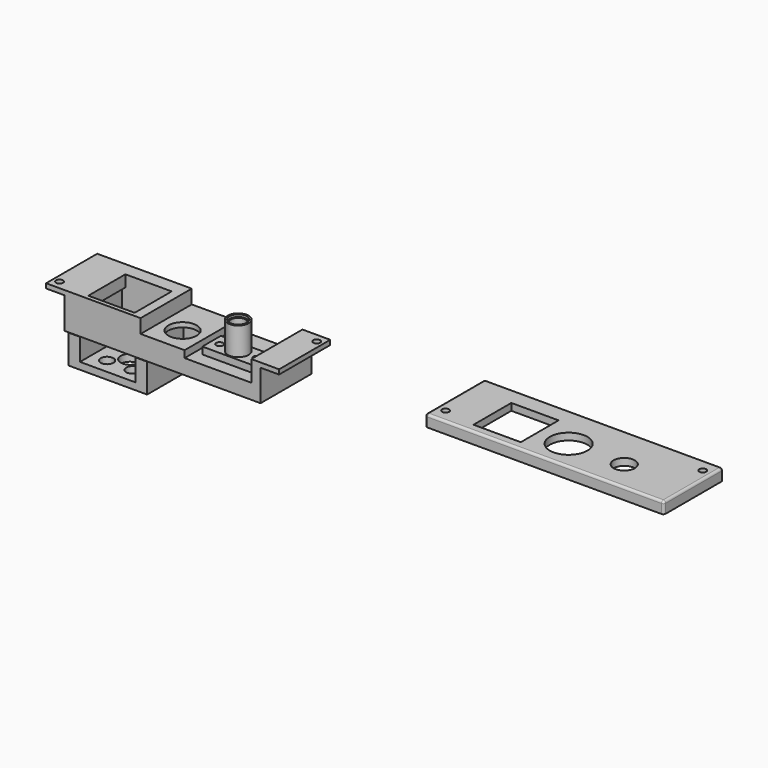
from build123d import *

# Parameters (mm, degrees)
F0_W      = 84.6
F0_H      = 27.6
F0_R      = 1.2
F0_R_2    = 3.1
F1_DEPTH  = 1.5
F2_W      = 103
F2_H      = 32
F2_R      = 1.5
F2_W_2    = 20.4
F2_H_2    = 20.4
F2_R_2    = 8.1
F2_R_3    = 4.6
F3_DEPTH  = 5
F4_W      = 101
F4_H      = 30
F5_DEPTH  = 2
F6_R      = 1
F7_W      = 8
F7_H      = 2
F8_DEPTH  = 27.6
F9_D      = 3
F9_DEPTH  = 5
F9_START  = 8.5
F9_TIP    = 0.9012909285
F10_W     = 23
F10_H     = 10
F10_R     = 1.5
F11_DEPTH = 3
F12_R     = 4.5
F13_DEPTH = 12
F14_R     = 3.1
F15_DEPTH = 25
F16_W     = 19
F16_H     = 27.6
F17_DEPTH = 3
F18_D     = 12.2
F18_DEPTH = 5
F18_TIP   = 3.6652497761
F19_R     = 3.75
F20_DEPTH = 1
F21_W     = 30.8
F21_H     = 9
F21_W_2   = 2
F21_W_3   = 84.6
F21_H_2   = 5
F22_DEPTH = 27.6
F23_W     = 20
F23_H     = 20
F24_DEPTH = 25
F25_W     = 1.5
F25_H     = 20
F26_DEPTH = 10.5
F27_W     = 13
F27_H     = 17
F28_DEPTH = 7.5
F30_W     = 34
F30_H     = 24
F31_DEPTH = 12.5
F32_W     = 24
F32_H     = 9.5
F33_DEPTH = 25
F34_R     = 4
F34_R_2   = 1.6
F34_R_3   = 2.75
F35_DEPTH = 25
F36_R     = 1.2
F37_DEPTH = 8
F38_DEPTH = 25


with BuildPart() as f1:
    # F0 (on Top) → F1 (new body)
    with BuildSketch(Plane.XY):
        Rectangle(F0_W, F0_H)
        with Locations((16, -3)):
            Circle(F0_R, mode=Mode.SUBTRACT)
        with Locations((24, -3)):
            Circle(F0_R_2, mode=Mode.SUBTRACT)
        with Locations((32, -3)):
            Circle(F0_R, mode=Mode.SUBTRACT)
    extrude(amount=F1_DEPTH)

    # F7 (on face) → F8 (join)
    with BuildSketch(Plane.XZ.offset(13.8)):
        Polygon((-42.3, 8.5), (-42.3, 1.5), (-40.3, 1.5), (-40.3, 10.5), (-50.3, 10.5), (-50.3, 8.5), align=None)
        Polygon((42.3, 8.5), (42.3, 10.5), (40.3, 10.5), (40.3, 1.5), (42.3, 1.5), align=None)
        with Locations((46.3, 9.5)):
            Rectangle(F7_W, F7_H)
    extrude(amount=-F8_DEPTH)

    # F9
    # its depths count from where the whole tool has entered the part; down to there all is cleared
    with Locations(Plane(origin=(0, 0, 0), x_dir=(1, 0, 0), z_dir=(0, 0, -1))):
        with Locations((-47.5, 10), (47.5, -10)):
            Hole(F9_D / 2, depth=F9_START)
    with Locations(Plane(origin=(0, 0, 0), x_dir=(1, 0, 0), z_dir=(0, 0, -1)).offset(-F9_START)):
        with Locations((-47.5, 10), (47.5, -10)):
            Hole(F9_D / 2, depth=F9_DEPTH)
            with Locations((0, 0, -(F9_DEPTH + F9_TIP / 2))):  # 118° drill point
                Cone(0, F9_D / 2, F9_TIP, mode=Mode.SUBTRACT)

    # F16 (on face) → F17 (join)
    with BuildSketch(Plane.XY.offset(1.5)):
        Rectangle(F16_W, F16_H)
    extrude(amount=F17_DEPTH)

    # F18
    with Locations(Plane(origin=(0, 0, 0), x_dir=(1, 0, 0), z_dir=(0, 0, -1))):
        with Locations((0, 3)):
            Hole(F18_D / 2, depth=F18_DEPTH)
            with Locations((0, 0, -(F18_DEPTH + F18_TIP / 2))):  # 118° drill point
                Cone(0, F18_D / 2, F18_TIP, mode=Mode.SUBTRACT)

    # F21 (on face) → F22 (join)
    with BuildSketch(Plane.XZ.offset(13.8)):
        with Locations((-24.9, 6)):
            Rectangle(F21_W, F21_H)
        with Locations((39.3, 6)):
            Rectangle(F21_W_2, F21_H)
        with Locations((0, -2.5)):
            Rectangle(F21_W_3, F21_H_2)
    extrude(amount=-F22_DEPTH)

    # F23 (on face) → F24 (cut)
    with BuildSketch(Plane.XY.offset(10.5)):
        with Locations((-23.5, -2)):
            Rectangle(F23_W, F23_H)
    extrude(amount=-F24_DEPTH, mode=Mode.SUBTRACT)

    # F25 (on face) → F26 (cut)
    with BuildSketch(Plane(origin=(0, 0, -5), x_dir=(1, 0, 0), z_dir=(0, 0, -1))):
        with Locations((-34.25, 2)):
            Rectangle(F25_W, F25_H)
        with Locations((-12.75, 2)):
            Rectangle(F25_W, F25_H)
    extrude(amount=-F26_DEPTH, mode=Mode.SUBTRACT)

    # F27 (on face) → F28 (cut)
    with BuildSketch(Plane(origin=(0, 0, -5), x_dir=(1, 0, 0), z_dir=(0, 0, -1))):
        with Locations((0, 3)):
            Rectangle(F27_W, F27_H)
    extrude(amount=-F28_DEPTH, mode=Mode.SUBTRACT)

    # F36 (on face) → F37 (cut)
    with BuildSketch(Plane(origin=(0, 0, -5), x_dir=(1, 0, 0), z_dir=(0, 0, -1))):
        with Locations((-38, 9.5)):
            Circle(F36_R)
        with Locations((-38, -5.5)):
            Circle(F36_R)
        with Locations((-9, 9.5)):
            Circle(F36_R)
        with Locations((-9, -5.5)):
            Circle(F36_R)
    extrude(amount=-F37_DEPTH, mode=Mode.SUBTRACT)

    # F38 (cut): faces of the model
    f38_faces = [f1.faces().sort_by_distance(p)[0] for p in [
        (16, -3, 0),
        (24, -3, 0),
        (32, -3, 0),
    ]]
    extrude(f38_faces, amount=-F38_DEPTH, mode=Mode.SUBTRACT)


with BuildPart() as f3:
    # F2 (on Top) → F3 (new body)
    with BuildSketch(Plane.XY):
        with Locations((153.8635194302, 16)):
            Rectangle(F2_W, F2_H)
        with Locations((106.3635194302, 6)):
            Circle(F2_R, mode=Mode.SUBTRACT)
        with Locations((130.3635194302, 14)):
            Rectangle(F2_W_2, F2_H_2, mode=Mode.SUBTRACT)
        with Locations((153.8635194302, 13)):
            Circle(F2_R_2, mode=Mode.SUBTRACT)
        with Locations((177.8635194302, 13)):
            Circle(F2_R_3, mode=Mode.SUBTRACT)
        with Locations((201.3635194302, 26)):
            Circle(F2_R, mode=Mode.SUBTRACT)
    extrude(amount=F3_DEPTH)

    # F4 (on face) → F5 (cut)
    with BuildSketch(Plane(origin=(0, 0, 0), x_dir=(1, 0, 0), z_dir=(0, 0, -1))):
        with Locations((153.8635194302, -16)):
            Rectangle(F4_W, F4_H)
    extrude(amount=-F5_DEPTH, mode=Mode.SUBTRACT)

    # F6
    f6_edges = [f3.edges().sort_by_distance(p)[0] for p in [
        (102.363519, 16, 5),
        (153.863519, 32, 5),
        (153.863519, 0, 5),
        (205.363519, 16, 5),
        (205.363519, 32, 2.5),
        (205.363519, 0, 2.5),
        (102.363519, 32, 2.5),
        (102.363519, 0, 2.5),
    ]]
    fillet(f6_edges, radius=F6_R)


with BuildPart() as f11:
    # F10 (on face) → F11 (new body)
    with BuildSketch(Plane.XY.offset(1.5)):
        with Locations((24, -3)):
            Rectangle(F10_W, F10_H)
        with Locations((16, -3)):
            Circle(F10_R, mode=Mode.SUBTRACT)
        with Locations((32, -3)):
            Circle(F10_R, mode=Mode.SUBTRACT)
    extrude(amount=F11_DEPTH)

    # F12 (on face) → F13 (join)
    with BuildSketch(Plane.XY.offset(4.5)):
        with Locations((24, -3)):
            Circle(F12_R)
    extrude(amount=F13_DEPTH)

    # F14 (on face) → F15 (cut)
    with BuildSketch(Plane.XY.offset(16.5)):
        with Locations((24, -3)):
            Circle(F14_R)
    extrude(amount=-F15_DEPTH, mode=Mode.SUBTRACT)

    # F19 (on face) → F20 (cut)
    with BuildSketch(Plane.XY.offset(16.5)):
        with Locations((24, -3)):
            Circle(F19_R)
    extrude(amount=-F20_DEPTH, mode=Mode.SUBTRACT)


with BuildPart() as f31:
    # F30 (on offset) → F31 (new body)
    with BuildSketch(Plane(origin=(0, 0, -17.5), x_dir=(1, 0, 0), z_dir=(0, 0, -1))):
        with Locations((-23.5, 2)):
            Rectangle(F30_W, F30_H)
    extrude(amount=-F31_DEPTH)

    # F32 (on face) → F33 (cut)
    with BuildSketch(Plane.XZ.offset(14)):
        with Locations((-23.5, -9.75)):
            Rectangle(F32_W, F32_H)
    extrude(amount=-F33_DEPTH, mode=Mode.SUBTRACT)

    # F34 (on face) → F35 (cut)
    with BuildSketch(Plane(origin=(0, 0, -17.5), x_dir=(1, 0, 0), z_dir=(0, 0, -1))):
        with Locations((-23.5, 2)):
            Circle(F34_R)
        with Locations((-38, 9.5)):
            Circle(F34_R_2)
        with Locations((-38, -5.5)):
            Circle(F34_R_2)
        with Locations((-9, 9.5)):
            Circle(F34_R_2)
        with Locations((-9, -5.5)):
            Circle(F34_R_2)
        with Locations((-29, 7.5)):
            Circle(F34_R_3)
        with Locations((-18, 7.5)):
            Circle(F34_R_3)
        with Locations((-29, -3.5)):
            Circle(F34_R_3)
        with Locations((-18, -3.5)):
            Circle(F34_R_3)
    extrude(amount=-F35_DEPTH, mode=Mode.SUBTRACT)


solid = Compound([f1.part, f3.part, f11.part, f31.part])
